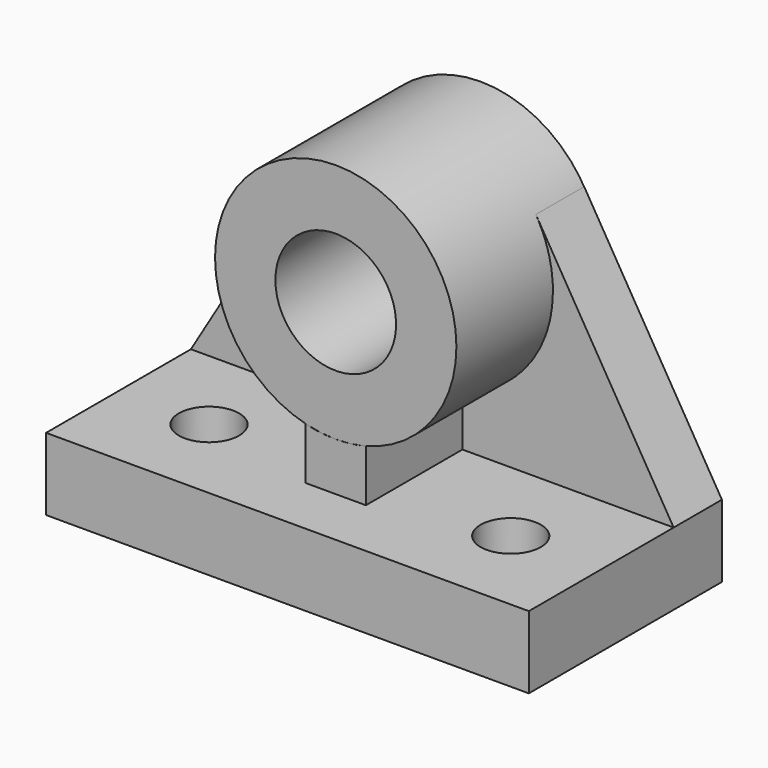
from build123d import *

# Parameters (mm, degrees)
F0_W     = 80
F0_H     = 40
F0_R     = 5
F1_DEPTH = 12
F2_R     = 20
F2_R_2   = 10
F3_DEPTH = 30
F5_DEPTH = 10
F7_DEPTH = 25


with BuildPart() as f1:
    # F0 (on Top) → F1 (new body)
    with BuildSketch(Plane.XY):
        Rectangle(F0_W, F0_H)
        with Locations((-25, -5)):
            Circle(F0_R, mode=Mode.SUBTRACT)
        with Locations((25, -5)):
            Circle(F0_R, mode=Mode.SUBTRACT)
    extrude(amount=F1_DEPTH)

    # F6 (on face) → F7 (join)
    with BuildSketch(Plane.XZ.offset(10)):
        with BuildLine():
            Line((0, 12), (5, 12))
            Line((5, 12), (5, 20.635083269))
            ThreePointArc((5, 20.635083269), (2.5200858497, 20.1594060747), (0, 20))
            Line((0, 20), (0, 12))
        make_face()
        with BuildLine():
            Line((-5, 20.635083269), (-5, 12))
            Line((-5, 12), (0, 12))
            Line((0, 12), (0, 20))
            ThreePointArc((0, 20), (-2.5200858497, 20.1594060747), (-5, 20.635083269))
        make_face()
    extrude(amount=-F7_DEPTH)


with BuildPart() as f3:
    # F2 (on face) → F3 (new body)
    with BuildSketch(Plane(origin=(0, 20, 0), x_dir=(-1, 0, 0), z_dir=(0, 1, 0))):
        with Locations((0, 40)):
            Circle(F2_R)
        with Locations((0, 40)):
            Circle(F2_R_2, mode=Mode.SUBTRACT)
    extrude(amount=-F3_DEPTH)


with BuildPart() as f5:
    # F4 (on face) → F5 (new body)
    with BuildSketch(Plane(origin=(0, 20, 0), x_dir=(-1, 0, 0), z_dir=(0, 1, 0))):
        with BuildLine():
            Line((-17.1743221847, 50.2490320273), (-40, 12))
            Line((-40, 12), (40, 12))
            Line((40, 12), (17.1743222859, 50.2490318576))
            ThreePointArc((17.1743222859, 50.2490318576), (19.2806437356, 45.3157104079), (20, 40))
            ThreePointArc((20, 40), (-5.3157105031, 20.7193562906), (-17.1743221847, 50.2490320273))
        make_face()
    extrude(amount=-F5_DEPTH)


solid = Compound([f1.part, f3.part, f5.part])
